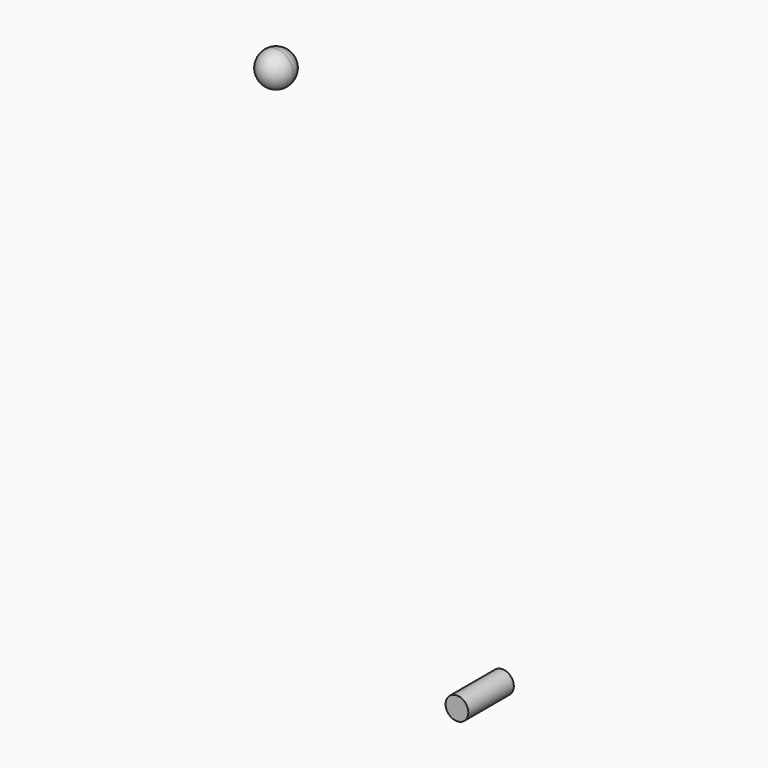
from build123d import *

# Parameters (mm, degrees)
F0_R     = 1.27
F1_DEPTH = 6.35
F2_DEPTH = 3.81
F0_R_2   = 1.905
F3_R     = 1.90499


# Not quite as in the source:
# - a fillet or chamfer is up to 0.001 mm smaller than in the source, because OpenCascade refuses the exact size


with BuildPart() as f1:
    # F0 (on Front) → F1 (new body)
    with BuildSketch(Plane.XZ):
        with Locations((-37.3650640249, -26.2328255922)):
            Circle(F0_R)
    extrude(amount=F1_DEPTH)

    # F0 (on Front) → F2 (join)
    with BuildSketch(Plane.XZ):
        with Locations((-37.3650640249, -26.2328255922)):
            Circle(F0_R)
    extrude(amount=F2_DEPTH)


with BuildPart() as f2:
    # F0 (on Front) → F2, piece 2 (new body)
    with BuildSketch(Plane.XZ):
        with Locations((-61.1126385629, 27.1582473069)):
            Circle(F0_R_2)
    extrude(amount=F2_DEPTH)

    # F3 (radius 1.905 in the source; OpenCascade refuses exactly that, so slightly less here)
    f3_edges = [f2.edges().sort_by_distance(p)[0] for p in [
        (-63.017639, 0, 27.158247),
        (-63.017639, -3.81, 27.158247),
    ]]
    fillet(f3_edges, radius=F3_R)


solid = Compound([f1.part, f2.part])
